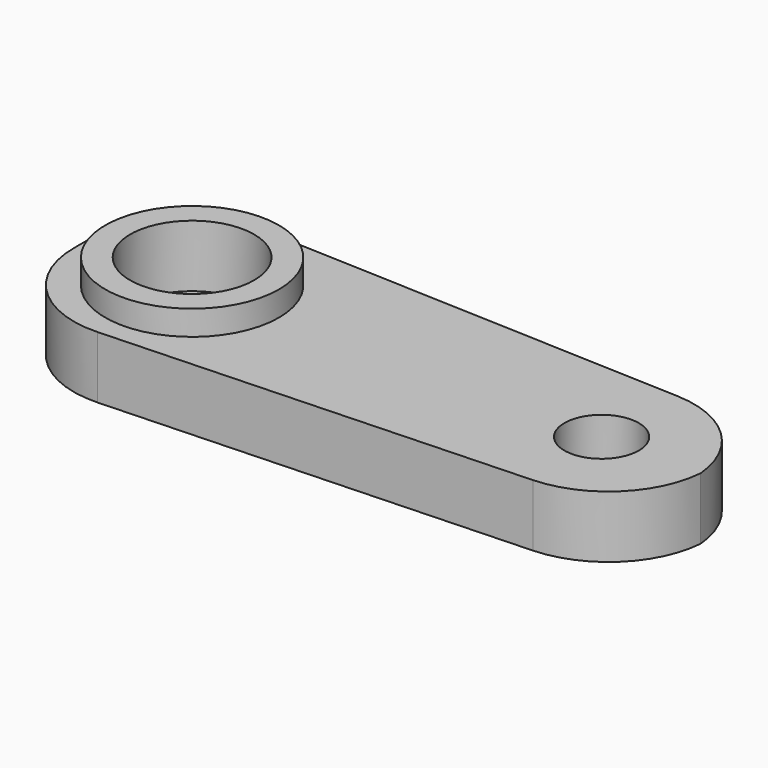
from build123d import *

# Parameters (mm, degrees)
F0_R        = 2.5
F0_R_2      = 1.5
F1_DEPTH    = 2.5
F2_T1_DEPTH = 21.7159936051
F2_T3_DEPTH = 23.3159936051
F3_R        = 3.5
F3_R_2      = 2.5
F4_DEPTH    = 1
F5_R        = 2.5
F5_R_2      = 1.1
F6_DEPTH    = 1


# Not quite as in the source:
# - a fillet or chamfer that OpenCascade refuses, or shapes differently, is made with other operations: its cross-section is extruded or revolved along the edge and cut away or added


with BuildPart() as f1:
    # F0 (on Top) → F1 (new body)
    with BuildSketch(Plane.XY):
        Polygon((25, -12), (0, -11), (0, -20), (25, -19), align=None)
        with Locations((4.5, -15.5)):
            Circle(F0_R, mode=Mode.SUBTRACT)
        with Locations((21, -15.5)):
            Circle(F0_R_2, mode=Mode.SUBTRACT)
    extrude(amount=F1_DEPTH)

    # F2: fillet of radius 4 on 4 edges, made by hand

    # F2_s2 → F2_t1 (cut)
    with BuildSketch(Plane.XY.offset(-9.6079968026)):
        with BuildLine():
            ThreePointArc((21.1598721534, -11.8463948861), (23.8843966972, -13.0718712966), (25, -15.843198721))
            Line((25, -15.843198721), (25, -12))
            Line((25, -12), (21.1598721534, -11.8463948861))
        make_face()
        with BuildLine():
            ThreePointArc((21.1598721534, -19.1536051139), (23.8843966972, -17.9281287034), (25, -15.156801279))
            Line((25, -15.156801279), (25, -19))
            Line((25, -19), (21.1598721534, -19.1536051139))
        make_face()
    extrude(amount=F2_T1_DEPTH, mode=Mode.SUBTRACT)

    # F2_s4 → F2_t3 (cut)
    with BuildSketch(Plane.XY.offset(-10.4079968026)):
        with BuildLine():
            ThreePointArc((4.1598721534, -11.1663948861), (1.2286725756, -12.2788020238), (0, -15.163198721))
            Line((0, -15.163198721), (0, -11))
            Line((0, -11), (4.1598721534, -11.1663948861))
        make_face()
        with BuildLine():
            ThreePointArc((0, -15.836801279), (1.2286725756, -18.7211979762), (4.1598721534, -19.8336051139))
            Line((4.1598721534, -19.8336051139), (0, -20))
            Line((0, -20), (0, -15.836801279))
        make_face()
    extrude(amount=F2_T3_DEPTH, mode=Mode.SUBTRACT)

    # F3 (on face) → F4 (join)
    with BuildSketch(Plane.XY.offset(2.5)):
        with Locations((4.5, -15.5)):
            Circle(F3_R)
        with Locations((4.5, -15.5)):
            Circle(F3_R_2, mode=Mode.SUBTRACT)
    extrude(amount=F4_DEPTH)

    # F5 (on Top) → F6 (join)
    with BuildSketch(Plane.XY):
        with Locations((4.5, -15.5)):
            Circle(F5_R)
        with Locations((4.5, -15.5)):
            Circle(F5_R_2, mode=Mode.SUBTRACT)
    extrude(amount=F6_DEPTH)


solid = f1.part
